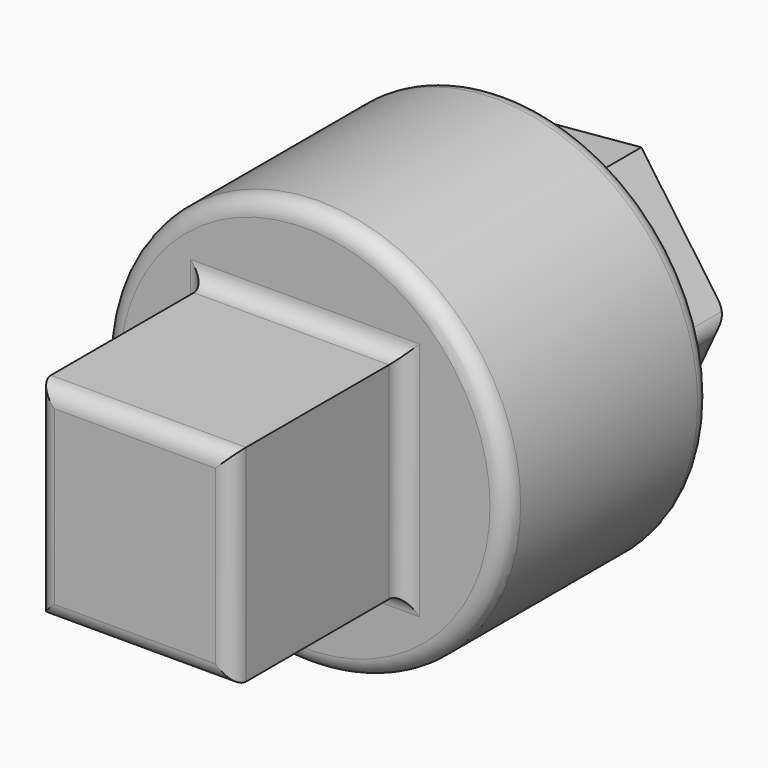
from build123d import *

# Parameters (mm, degrees)
F0_R     = 60.3524841782
F1_DEPTH = 76.2
F3_W     = 58.3018623292
F3_H     = 61.5784339607
F4_DEPTH = 63.5
F7_DEPTH = 25.4
F8_F1_R  = 5.08
F8_F2_R  = 5.08
F9_R     = 5.08
F10_R    = 5.08


with BuildPart() as f1:
    # F0 (on Front) → F1 (new body)
    with BuildSketch(Plane.XZ):
        Circle(F0_R)
    extrude(amount=F1_DEPTH)

    # F3 (on face) → F4 (join)
    with BuildSketch(Plane.XZ.offset(76.2)):
        Rectangle(F3_W, F3_H)
    extrude(amount=F4_DEPTH)

    # F6 (on face) → F7 (join)
    with BuildSketch(Plane(origin=(0, 0, 0), x_dir=(-1, 0, 0), z_dir=(0, 1, 0))):
        Polygon((19.1640303054, -41.3700494554), (45.4095289369, -4.0884876443), (26.2454986315, 37.2815618111), (-19.1640303054, 41.3700494554), (-45.4095289369, 4.0884876443), (-26.2454986315, -37.2815618111), align=None)
    extrude(amount=F7_DEPTH)

    # F8: fillet of radius 5.08 on 4 edges, made by hand

    # F8_f1
    f8_f1_edges = [f1.edges().sort_by_distance(p)[0] for p in [
        (45.4095289369, 12.7, 4.0884876443),
        (26.2454986315, 12.7, -37.2815618111),
        (35.8275137842, 25.4, -16.5965370834),
    ]]
    fillet(f8_f1_edges, radius=F8_F1_R)

    # F8_f2
    f8_f2_edges = [f1.edges().sort_by_distance(p)[0] for p in [
        (35.8275137842, 0, -16.5965370834),
        (44.6268163137, 0, 4.0180154116),
        (25.7931115761, 0, -36.6389489119),
    ]]
    fillet(f8_f2_edges, radius=F8_F2_R)

    # F9
    f9_edges = [f1.edges().sort_by_distance(p)[0] for p in [
        (0, -139.7, -30.789217),
        (29.150931, -139.7, 0),
        (0, -139.7, 30.789217),
        (-29.150931, -139.7, 0),
        (-60.352484, -76.2, 0),
        (0, -76.2, -30.789217),
        (29.150931, -76.2, 0),
        (0, -76.2, 30.789217),
        (-29.150931, -76.2, 0),
    ]]
    fillet(f9_edges, radius=F9_R)

    # F10
    f10_edges = [f1.edges().sort_by_distance(p)[0] for p in [
        (-60.352484, 0, 0),
    ]]
    fillet(f10_edges, radius=F10_R)


solid = f1.part
